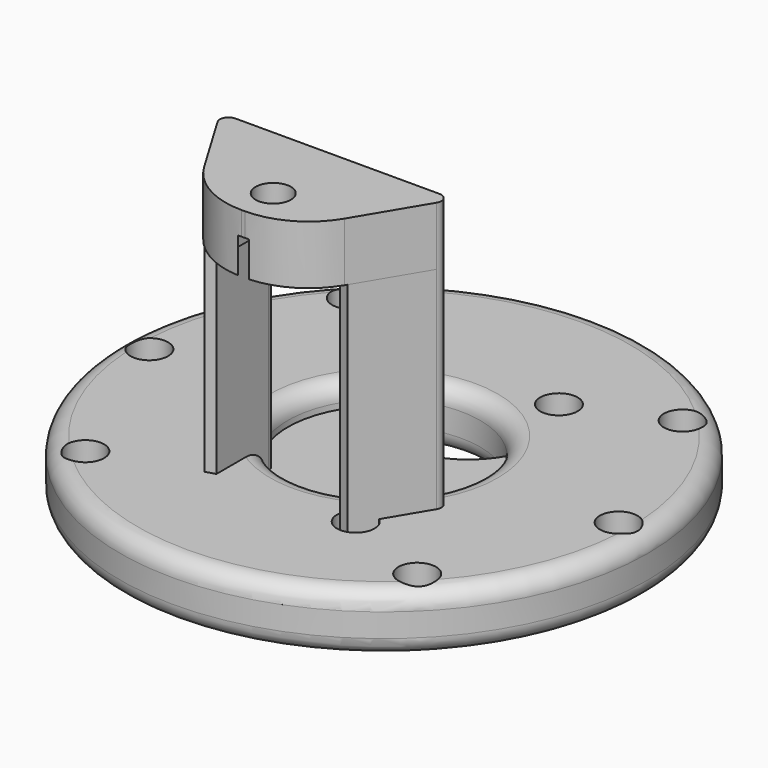
from build123d import *

# Parameters (mm, degrees)
F0_R     = 6.6
F1_DEPTH = 3
F3_DEPTH = 20
F4_R     = 1.5
F5_DEPTH = 5
F6_R     = 1.5
F7_DEPTH = 3
F8_R     = 22.5
F8_R_2   = 1.6
F8_R_3   = 8.2
F9_DEPTH = 5


# Not quite as in the source:
# - a fillet or chamfer that OpenCascade refuses, or shapes differently, is made with other operations: its cross-section is extruded or revolved along the edge and cut away or added


with BuildPart() as f1:
    # F0 (on Top) → F1 (new body)
    with BuildSketch(Plane.XY):
        with BuildLine():
            Line((10, -4.9520083861), (10, 3.0479916139))
            ThreePointArc((10, 3.0479916139), (0, 20.6280349051), (-10, 3.0479916139))
            Line((-10, 3.0479916139), (-10, -4.9520083861))
            Line((-10, -4.9520083861), (-6.0899698972, -11.5))
            ThreePointArc((-6.0899698972, -11.5), (0, -10.5502563408), (6.0899698972, -11.5))
            Line((6.0899698972, -11.5), (10, -4.9520083861))
        make_face()
        with Locations((0, 8.9938791938)):
            Circle(F0_R, mode=Mode.SUBTRACT)
    extrude(amount=F1_DEPTH)

    # F2 (on face) → F3 (join)
    with BuildSketch(Plane.XY.offset(3)):
        with BuildLine():
            Line((-6.0187778734, -4.9520083861), (-8.694429646, -4.9520083861))
            ThreePointArc((-8.694429646, -4.9520083861), (-9.33888075, -5.3272492941), (-9.3306530777, -6.0729404298))
            Line((-9.3306530777, -6.0729404298), (-6.0899698972, -11.5))
            ThreePointArc((-6.0899698972, -11.5), (-5.6851384444, -11.375293476), (-5.2777566353, -11.259188851))
            Line((-5.2777566353, -11.259188851), (-5.2777566353, -5.6930296241))
            ThreePointArc((-5.2777566353, -5.6930296241), (-5.494796731, -5.1690484817), (-6.0187778734, -4.9520083861))
        make_face()
        with BuildLine():
            Line((5.2777566353, -5.6930296241), (5.2777566353, -11.259188851))
            ThreePointArc((5.2777566353, -11.259188851), (5.6851384444, -11.375293476), (6.0899698972, -11.5))
            Line((6.0899698972, -11.5), (9.3306530777, -6.0729404298))
            ThreePointArc((9.3306530777, -6.0729404298), (9.33888075, -5.3272492941), (8.694429646, -4.9520083861))
            Line((8.694429646, -4.9520083861), (6.0187778734, -4.9520083861))
            ThreePointArc((6.0187778734, -4.9520083861), (5.494796731, -5.1690484817), (5.2777566353, -5.6930296241))
        make_face()
    extrude(amount=F3_DEPTH)

    # F4 (on face) → F5 (join)
    with BuildSketch(Plane.XY.offset(23)):
        with BuildLine():
            Line((8.694429646, -4.9520083861), (-6.0187778734, -4.9520083861))
            ThreePointArc((-6.0187778734, -4.9520083861), (-5.494796731, -5.1690484817), (-5.2777566353, -5.6930296241))
            Line((-5.2777566353, -5.6930296241), (-5.2777566353, -11.259188851))
            ThreePointArc((-5.2777566353, -11.259188851), (-5.6851384444, -11.375293476), (-6.0899698972, -11.5))
            Line((-6.0899698972, -11.5), (-5.9729271999, -11.6960073402))
            ThreePointArc((-5.9729271999, -11.6960073402), (-3.4984984861, -14.1164281462), (-0.1517784325, -15))
            Line((-0.1517784325, -15), (0.1517784325, -15))
            ThreePointArc((0.1517784325, -15), (3.4984984861, -14.1164281462), (5.9729271999, -11.6960073402))
            Line((5.9729271999, -11.6960073402), (9.3306530777, -6.0729404298))
            ThreePointArc((9.3306530777, -6.0729404298), (9.33888075, -5.3272492941), (8.694429646, -4.9520083861))
        make_face()
        with Locations((0, -11.8)):
            Circle(F4_R, mode=Mode.SUBTRACT)
        with BuildLine():
            Line((-6.0187778734, -4.9520083861), (-8.694429646, -4.9520083861))
            ThreePointArc((-8.694429646, -4.9520083861), (-9.33888075, -5.3272492941), (-9.3306530777, -6.0729404298))
            Line((-9.3306530777, -6.0729404298), (-6.0899698972, -11.5))
            ThreePointArc((-6.0899698972, -11.5), (-5.6851384444, -11.375293476), (-5.2777566353, -11.259188851))
            Line((-5.2777566353, -11.259188851), (-5.2777566353, -5.6930296241))
            ThreePointArc((-5.2777566353, -5.6930296241), (-5.494796731, -5.1690484817), (-6.0187778734, -4.9520083861))
        make_face()
    extrude(amount=F5_DEPTH)

    # F6 (on face) → F7 (cut)
    with BuildSketch(Plane(origin=(0, 0, 23), x_dir=(1, 0, 0), z_dir=(0, 0, -1))):
        with BuildLine():
            Line((-0.4704129933, 14.9925085468), (-3, 13.5320508076))
            Line((-3, 13.5320508076), (-3, 10.0679491924))
            Line((-3, 10.0679491924), (0, 8.3358983849))
            Line((0, 8.3358983849), (3, 10.0679491924))
            Line((3, 10.0679491924), (3, 13.5320508076))
            Line((3, 13.5320508076), (0.4704129933, 14.9925085468))
            ThreePointArc((0.4704129933, 14.9925085468), (0.31113974, 14.998126878), (0.1517784325, 15))
            Line((0.1517784325, 15), (-0.1517784325, 15))
            ThreePointArc((-0.1517784325, 15), (-0.3111397399, 14.998126878), (-0.4704129933, 14.9925085468))
        make_face()
        with Locations((0, 11.8)):
            Circle(F6_R, mode=Mode.SUBTRACT)
    extrude(amount=-F7_DEPTH, mode=Mode.SUBTRACT)


with BuildPart() as f9:
    # F8 (on Top) → F9 (new body)
    with BuildSketch(Plane.XY):
        Circle(F8_R)
        with Locations((-14.1421356237, -14.1421356237)):
            Circle(F8_R_2, mode=Mode.SUBTRACT)
        with Locations((14.1421356237, -14.1421356237)):
            Circle(F8_R_2, mode=Mode.SUBTRACT)
        with Locations((6.25, -10.8253175473)):
            Circle(F8_R_2, mode=Mode.SUBTRACT)
        with Locations((-20, 0)):
            Circle(F8_R_2, mode=Mode.SUBTRACT)
        with Locations((-12.5, 0)):
            Circle(F8_R_2, mode=Mode.SUBTRACT)
        with Locations((-14.1421356237, 14.1421356237)):
            Circle(F8_R_2, mode=Mode.SUBTRACT)
        Circle(F8_R_3, mode=Mode.SUBTRACT)
        with Locations((6.25, 10.8253175473)):
            Circle(F8_R_2, mode=Mode.SUBTRACT)
        with Locations((20, 0)):
            Circle(F8_R_2, mode=Mode.SUBTRACT)
        with Locations((14.1421356237, 14.1421356237)):
            Circle(F8_R_2, mode=Mode.SUBTRACT)
    extrude(amount=F9_DEPTH)

    # F10: fillet of radius 1.5 on 1 edges, made by hand

    # F10_s1 → F10_t2 (revolve, cut)
    with BuildSketch(Plane.XZ):
        with BuildLine():
            ThreePointArc((22.5, 3.5), (22.0606601718, 4.5606601718), (21, 5))
            Line((21, 5), (22.5, 5))
            Line((22.5, 5), (22.5, 3.5))
        make_face()
    revolve(axis=Axis((0, 0, 5), (0, 0, 1)), mode=Mode.SUBTRACT)

    # F11: fillet of radius 1.5 on 3 edges, made by hand

    # F11_s1 → F11_t2 (revolve, cut)
    with BuildSketch(Plane.XZ):
        with BuildLine():
            ThreePointArc((22.5, 1.5), (22.0606601718, 0.4393398282), (21, 0))
            Line((21, 0), (22.5, 0))
            Line((22.5, 0), (22.5, 1.5))
        make_face()
    revolve(axis=Axis((0, 0, 0), (0, 0, 1)), mode=Mode.SUBTRACT)

    # F11_s3 → F11_t4 (revolve, cut)
    with BuildSketch(Plane.XZ):
        with BuildLine():
            ThreePointArc((9.7, 0), (8.6393398282, 0.4393398282), (8.2, 1.5))
            Line((8.2, 1.5), (8.2, 0))
            Line((8.2, 0), (9.7, 0))
        make_face()
    revolve(axis=Axis((0, 0, 0), (0, 0, 1)), mode=Mode.SUBTRACT)

    # F11_s5 → F11_t6 (revolve, cut)
    with BuildSketch(Plane.XZ):
        with BuildLine():
            ThreePointArc((8.2, 3.5), (8.6393398282, 4.5606601718), (9.7, 5))
            Line((9.7, 5), (8.2, 5))
            Line((8.2, 5), (8.2, 3.5))
        make_face()
    revolve(axis=Axis((0, 0, 5), (0, 0, 1)), mode=Mode.SUBTRACT)


solid = Compound([f1.part, f9.part])
